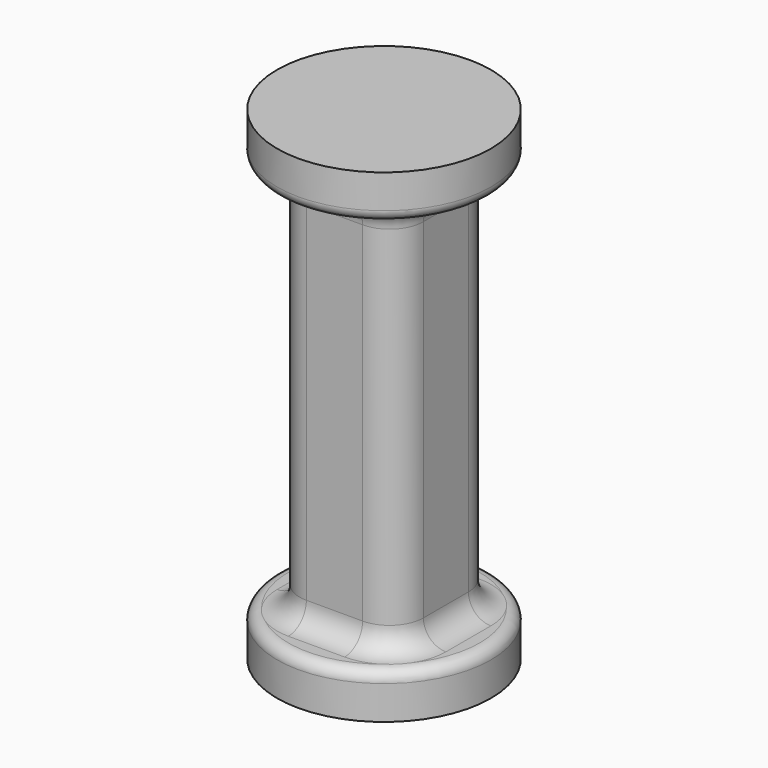
from build123d import *

# Parameters (mm, degrees)
F0_R     = 9.5
F1_DEPTH = 4
F2_W     = 11
F2_H     = 11
F3_DEPTH = 35
F6_R     = 3
F7_R     = 2


# Not quite as in the source:
# - a fillet or chamfer that OpenCascade refuses, or shapes differently, is made with other operations: its cross-section is extruded or revolved along the edge and cut away or added
# - a pattern or mirror of a feature is missing from the dataset's text; its kind, count and spacing are read off the source's solid


with BuildPart() as f1:
    # F0 (on Top) → F1 (new body)
    with BuildSketch(Plane.XY):
        Circle(F0_R)
    extrude(amount=F1_DEPTH)


with BuildPart() as f1_copies_1:
    # F1_copies: instance of F1
    add(f1.part.mirror(Plane.XY.offset(21.499996)))


with BuildPart() as f1_1:
    add(f1.part)

    add(f1_copies_1.part)  # F3 merges F1_copies_1
    # F2 (on face) → F3 (join)
    with BuildSketch(Plane.XY.offset(4)):
        Rectangle(F2_W, F2_H)
    extrude(amount=F3_DEPTH)

    # F6
    f6_edges = [f1_1.edges().sort_by_distance(p)[0] for p in [
        (5.5, -5.5, 21.499996),
        (5.5, 5.5, 21.499996),
        (-5.5, -5.5, 21.499996),
        (-5.5, 5.5, 21.499996),
    ]]
    fillet(f6_edges, radius=F6_R)

    # F7
    f7_edges = [f1_1.edges().sort_by_distance(p)[0] for p in [
        (0, 5.5, 4),
        (2.5, 5.5, 21.499996),
        (-2.5, 5.5, 21.499996),
        (0, 5.5, 38.999992),
        (4.62132, 4.62132, 4),
        (5.5, 0, 38.999992),
        (4.62132, 4.62132, 38.999992),
        (4.62132, -4.62132, 38.999992),
        (0, -5.5, 38.999992),
        (-4.62132, 4.62132, 38.999992),
        (-4.62132, -4.62132, 38.999992),
        (-5.5, 0, 38.999992),
        (5.5, 0, 4),
        (4.62132, -4.62132, 4),
        (0, -5.5, 4),
        (-4.62132, 4.62132, 4),
        (-4.62132, -4.62132, 4),
        (-5.5, 0, 4),
    ]]
    fillet(f7_edges, radius=F7_R)

    # F8: fillet of radius 1 on 2 edges, made by hand

    # F8_s1 → F8_t2 (revolve, cut)
    with BuildSketch(Plane.XZ):
        with BuildLine():
            ThreePointArc((8.5, 4), (9.2071067812, 3.7071067812), (9.5, 3))
            Line((9.5, 3), (9.5, 4))
            Line((9.5, 4), (8.5, 4))
        make_face()
    revolve(axis=Axis((0, 0, 4), (0, 0, 1)), mode=Mode.SUBTRACT)

    # F8_s3 → F8_t4 (revolve, cut)
    with BuildSketch(Plane.XZ):
        with BuildLine():
            ThreePointArc((8.5, 38.999992), (9.2071067812, 39.2928852188), (9.5, 39.999992))
            Line((9.5, 39.999992), (9.5, 38.999992))
            Line((9.5, 38.999992), (8.5, 38.999992))
        make_face()
    revolve(axis=Axis((0, 0, 38.999992), (0, 0, 1)), mode=Mode.SUBTRACT)


solid = f1_1.part
